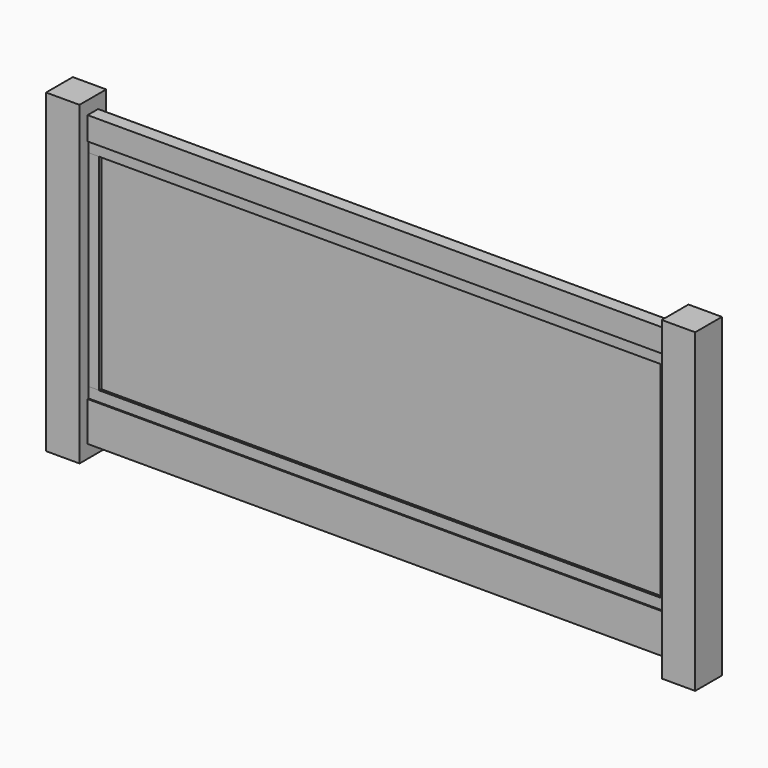
from build123d import *

# Parameters (mm, degrees)
F1_DEPTH      = 63.5
F1_DEPTH_BACK = 63.5
F0_W          = 2213
F0_H          = 150
F2_DEPTH      = 25
F2_DEPTH_BACK = 25
F0_H_2        = 88
F3_DEPTH      = 20
F3_DEPTH_BACK = 20
F0_W_2        = 40
F0_H_3        = 782
F0_W_3        = 2133
F4_DEPTH      = 10
F4_DEPTH_BACK = 10
F5_DEPTH      = 20
F5_DEPTH_BACK = 20


# Not quite as in the source:
# - a feature names something its author has since deleted; it is built from what else it names


with BuildPart() as f1:
    # F0 (on Front) → F1 (new body, two sides)
    with BuildSketch(Plane.XZ) as f1_sk:
        Polygon((-1106.5, -600), (-1106.5, -550), (-1106.5, -400), (-1106.5, -360), (-1106.5, 422), (-1106.5, 462), (-1106.5, 550), (-1106.5, 600), (-1233.5, 600), (-1233.5, -600), align=None)
    extrude(amount=F1_DEPTH)
    extrude(f1_sk.sketch, amount=-F1_DEPTH_BACK)


with BuildPart() as f1b:
    # F0 (on Front) → F1, piece 2 (new body, two sides)
    with BuildSketch(Plane.XZ) as f1_2_sk:
        Polygon((1106.5, -600), (1233.5, -600), (1233.5, 600), (1106.5, 600), (1106.5, 550), (1106.5, 462), (1106.5, 422), (1106.5, -360), (1106.5, -400), (1106.5, -550), align=None)
    extrude(amount=F1_DEPTH)
    extrude(f1_2_sk.sketch, amount=-F1_DEPTH_BACK)


with BuildPart() as f2:
    # F0 (on Front) → F2 (new body, two sides)
    with BuildSketch(Plane.XZ) as f2_sk:
        with Locations((0, -475)):
            Rectangle(F0_W, F0_H)
    extrude(amount=F2_DEPTH)
    extrude(f2_sk.sketch, amount=-F2_DEPTH_BACK)


with BuildPart() as f2b:
    # F0 (on Front) → F2, piece 2 (new body, two sides)
    with BuildSketch(Plane.XZ) as f2_2_sk:
        with Locations((0, 506)):
            Rectangle(F0_W, F0_H_2)
    extrude(amount=F2_DEPTH)
    extrude(f2_2_sk.sketch, amount=-F2_DEPTH_BACK)


with BuildPart() as f3:
    # F0 (on Front) → F3 (new body, two sides)
    with BuildSketch(Plane.XZ) as f3_sk:
        Polygon((1106.5, 422), (1106.5, 462), (-1106.5, 462), (-1106.5, 422), (-1066.5, 422), (1066.5, 422), align=None)
    extrude(amount=F3_DEPTH)
    extrude(f3_sk.sketch, amount=-F3_DEPTH_BACK)


with BuildPart() as f3b:
    # F0 (on Front) → F3, piece 2 (new body, two sides)
    with BuildSketch(Plane.XZ) as f3_2_sk:
        Polygon((-1106.5, -400), (1106.5, -400), (1106.5, -360), (1066.5, -360), (-1066.5, -360), (-1106.5, -360), align=None)
    extrude(amount=F3_DEPTH)
    extrude(f3_2_sk.sketch, amount=-F3_DEPTH_BACK)


with BuildPart() as f4:
    # F0 (on Front) → F4 (new body, two sides)
    with BuildSketch(Plane.XZ) as f4_sk:
        with Locations((-1086.5, 31)):
            Rectangle(F0_W_2, F0_H_3)
        with Locations((0, 31)):
            Rectangle(F0_W_3, F0_H_3)
        with Locations((1086.5, 31)):
            Rectangle(F0_W_2, F0_H_3)
    extrude(amount=F4_DEPTH)
    extrude(f4_sk.sketch, amount=-F4_DEPTH_BACK)


with BuildPart() as f5:
    # F0 (on Front) → F5 (new body, two sides)
    with BuildSketch(Plane.XZ) as f5_sk:
        with Locations((-1086.5, 31)):
            Rectangle(F0_W_2, F0_H_3)
    extrude(amount=F5_DEPTH)
    extrude(f5_sk.sketch, amount=-F5_DEPTH_BACK)


with BuildPart() as f5b:
    # F0 (on Front) → F5, piece 2 (new body, two sides)
    with BuildSketch(Plane.XZ) as f5_2_sk:
        with Locations((1086.5, 31)):
            Rectangle(F0_W_2, F0_H_3)
    extrude(amount=F5_DEPTH)
    extrude(f5_2_sk.sketch, amount=-F5_DEPTH_BACK)


solid = Compound([f1.part, f1b.part, f2.part, f2b.part, f3.part, f3b.part, f4.part, f5.part, f5b.part])
